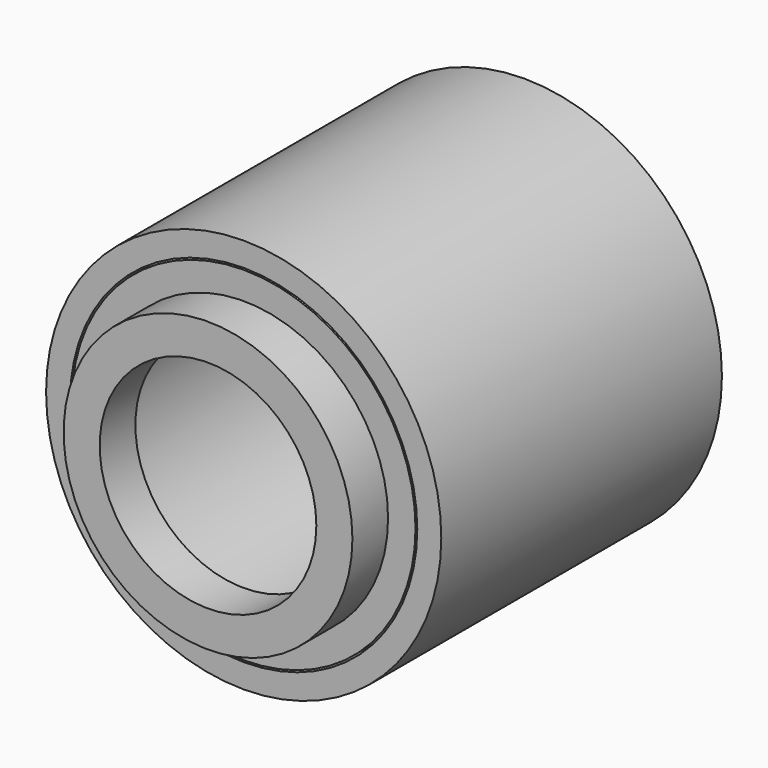
from build123d import *

# Parameters (mm, degrees)
F0_R     = 4.4329603323
F0_R_2   = 3.894738079
F1_DEPTH = 7.87
F0_R_3   = 3.855
F0_R_4   = 3.239330786
F0_R_5   = 2.43
F2_DEPTH = 1


# Not quite as in the source:
# - the program builds the solid bodies; features that only make, move or delete a surface that nothing else refers to are left out


with BuildPart() as f1:
    # F0 (on Front) → F1 (new body)
    with BuildSketch(Plane.XZ):
        Circle(F0_R)
        Circle(F0_R_2, mode=Mode.SUBTRACT)
    extrude(amount=-F1_DEPTH)


with BuildPart() as f1b:
    # F0 (on Front) → F1, piece 2 (new body)
    with BuildSketch(Plane.XZ):
        Circle(F0_R_3)
        Circle(F0_R_4, mode=Mode.SUBTRACT)
    extrude(amount=-F1_DEPTH)


with BuildPart() as f2:
    # F0 (on Front) → F2 (new body)
    with BuildSketch(Plane.XZ):
        Circle(F0_R_4)
        Circle(F0_R_5, mode=Mode.SUBTRACT)
    extrude(amount=F2_DEPTH)


solid = Compound([f1.part, f1b.part, f2.part])
